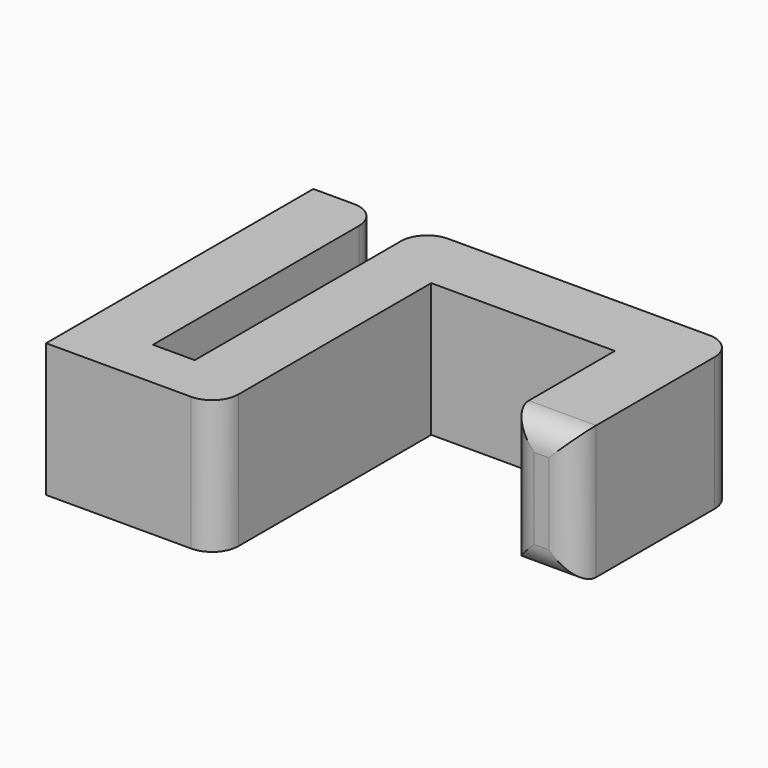
from build123d import *

# Parameters (mm, degrees)
F1_DEPTH     = 25.4
F2_R         = 5
F3_TEXT_SIZE = 24.2559612056
F4_DEPTH     = 2


# Not quite as in the source:
# - Text() gives the source's letters only with a copy of the font that has no kerning and outlines rounded to 1/6400 em; it was checked with that copy


with BuildPart() as f1:
    # F0 (on Top) → F1 (new body)
    with BuildSketch(Plane.XY):
        Polygon((0, 63.5), (0, 0), (32.5752518936, 0), (32.5752518936, 50.8), (67.4797778515, 50.8), (67.4797778515, 25.3516854542), (80.2734648196, 25.3516854542), (80.2734648196, 63.5), (20.6375, 63.5), (20.6375, 9.52754), (12.7, 9.52754), (12.7, 63.5), align=None)
    extrude(amount=F1_DEPTH)

    # F2
    f2_edges = [f1.edges().sort_by_distance(p)[0] for p in [
        (73.876621, 25.351685, 25.4),
        (73.876621, 25.351685, 0),
        (80.273465, 25.351685, 12.7),
        (67.479778, 25.351685, 12.7),
        (80.273465, 63.5, 12.7),
        (32.575252, 0, 12.7),
        (20.6375, 63.5, 12.7),
        (12.7, 63.5, 12.7),
    ]]
    fillet(f2_edges, radius=F2_R)

    # F3 (on face) → F4 (cut)
    with BuildSketch(Plane(origin=(0, 0, 0), x_dir=(0, -1, 0), z_dir=(-1, 0, 0))):
        with Locations((-61.9398709348, 4.7203872167)):
            Text('ABBY', F3_TEXT_SIZE, font='Open Sans', text_align=(TextAlign.LEFT, TextAlign.BOTTOM))
    extrude(amount=-F4_DEPTH, mode=Mode.SUBTRACT)


solid = f1.part
